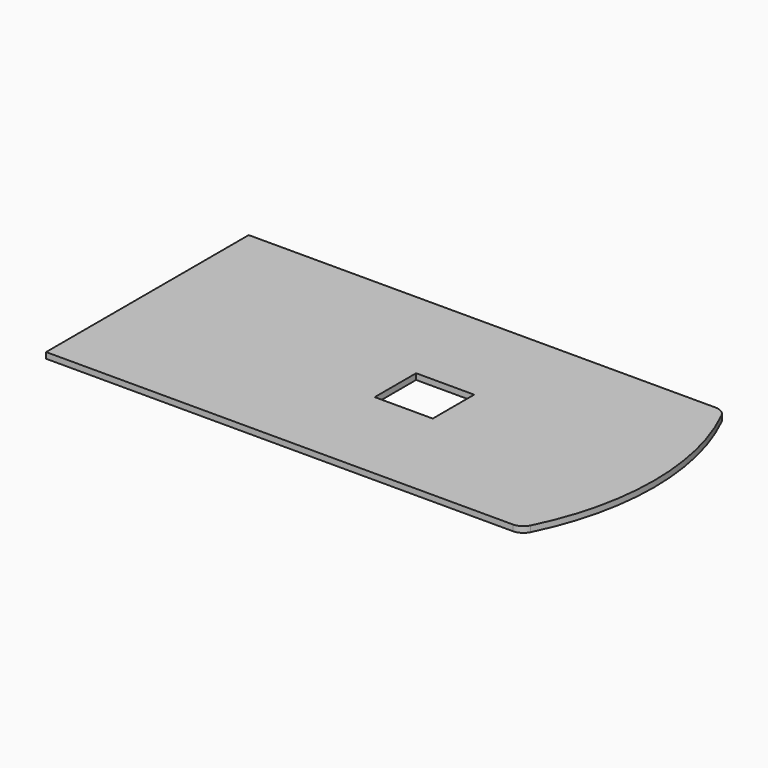
from build123d import *

# Parameters (mm, degrees)
F1_DEPTH = 28.575


# Not quite as in the source:
# - a feature names something its author has since deleted; it is built from what else it names


with BuildPart() as f1:
    # F0 (on Top) → F1 (new body)
    with BuildSketch(Plane.XY):
        with BuildLine():
            Line((1104.2429080596, 609.6), (-1143, 609.6))
            Line((-1143, 609.6), (-1143, 0))
            Line((-1143, 0), (50.8, 0))
            Line((50.8, 0), (50.8, 124.587))
            Line((50.8, 124.587), (330.2, 124.587))
            Line((330.2, 124.587), (330.2, 0))
            Line((330.2, 0), (1143, 0))
            Line((1143, 0), (1295.4, 0))
            ThreePointArc((1295.4, 0), (1261.3943180258, 294.8652818701), (1161.1626455885, 574.2494845361))
            ThreePointArc((1161.1626455885, 574.2494845361), (1137.7448313773, 600.0432213908), (1104.2429080596, 609.6))
        make_face()
        with BuildLine():
            Line((50.8, 0), (-1143, 0))
            Line((-1143, 0), (-1143, -609.6))
            Line((-1143, -609.6), (1104.2429080596, -609.6))
            ThreePointArc((1104.2429080596, -609.6), (1137.7448313773, -600.0432213908), (1161.1626455885, -574.2494845361))
            ThreePointArc((1161.1626455885, -574.2494845361), (1261.3943180258, -294.8652818701), (1295.4, 0))
            Line((1295.4, 0), (1143, 0))
            Line((1143, 0), (330.2, 0))
            Line((330.2, 0), (330.2, -124.587))
            Line((330.2, -124.587), (50.8, -124.587))
            Line((50.8, -124.587), (50.8, 0))
        make_face()
    extrude(amount=F1_DEPTH)


solid = f1.part
